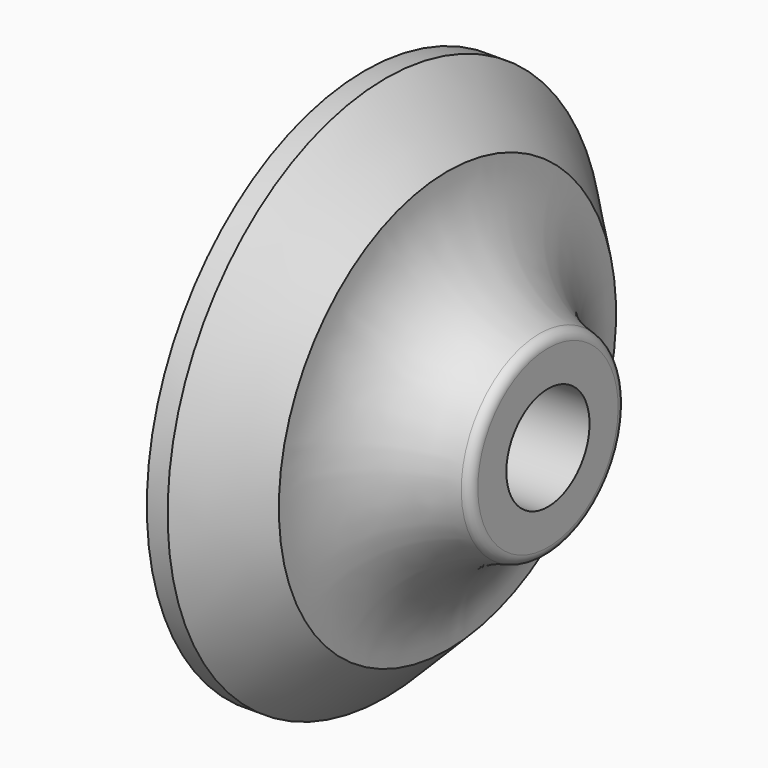
from build123d import *

# Parameters (mm, degrees)
F3_R     = 3.175
F4_DEPTH = 25.4
F5_R     = 3.81
F7_R     = 1.4732
F8_DEPTH = 1.905


# Not quite as in the source:
# - an extrude whose draft closes it to a point is written as a loft to that point


with BuildPart() as f1:
    # F0 (on Front) → F1 (revolve)
    with BuildSketch(Plane.XZ):
        with BuildLine():
            Line((-1.27, 16.637), (-1.27, 0))
            Line((-1.27, 0), (9.906, 0))
            Line((9.906, 0), (9.906, 5.3514806986))
            ThreePointArc((9.906, 5.3514806986), (9.7616470495, 5.7545817689), (9.3942189832, 5.9744109372))
            ThreePointArc((9.3942189832, 5.9744109372), (5.3425686191, 8.407770264), (3.7717075708, 12.8652924292))
            Line((3.7717075708, 12.8652924292), (0, 16.637))
            Line((0, 16.637), (-1.27, 16.637))
        make_face()
    revolve(axis=Axis((4.318, 0, 0), (1, 0, 0)))

    # F3 (on face) → F4 (cut)
    with BuildSketch(Plane(origin=(-1.27, 0, 0), x_dir=(0, -1, 0), z_dir=(-1, 0, 0))):
        Circle(F3_R)
    extrude(amount=-F4_DEPTH, mode=Mode.SUBTRACT)

    # F5 (on face) → F6 section 0
    with BuildSketch(Plane(origin=(-1.27, 0, 0), x_dir=(0, -1, 0), z_dir=(-1, 0, 0)), mode=Mode.PRIVATE) as f6_s0:
        Circle(F5_R)
    loft([f6_s0.sketch, Vertex(2.54, 0, 0)], ruled=True, mode=Mode.SUBTRACT)

    # F7 (on face) → F8 (cut)
    with BuildSketch(Plane(origin=(-1.27, 0, 0), x_dir=(0, -1, 0), z_dir=(-1, 0, 0))):
        with Locations((-8.255, 0)):
            Circle(F7_R)
        with Locations((8.255, 0)):
            Circle(F7_R)
    extrude(amount=-F8_DEPTH, mode=Mode.SUBTRACT)


solid = f1.part
